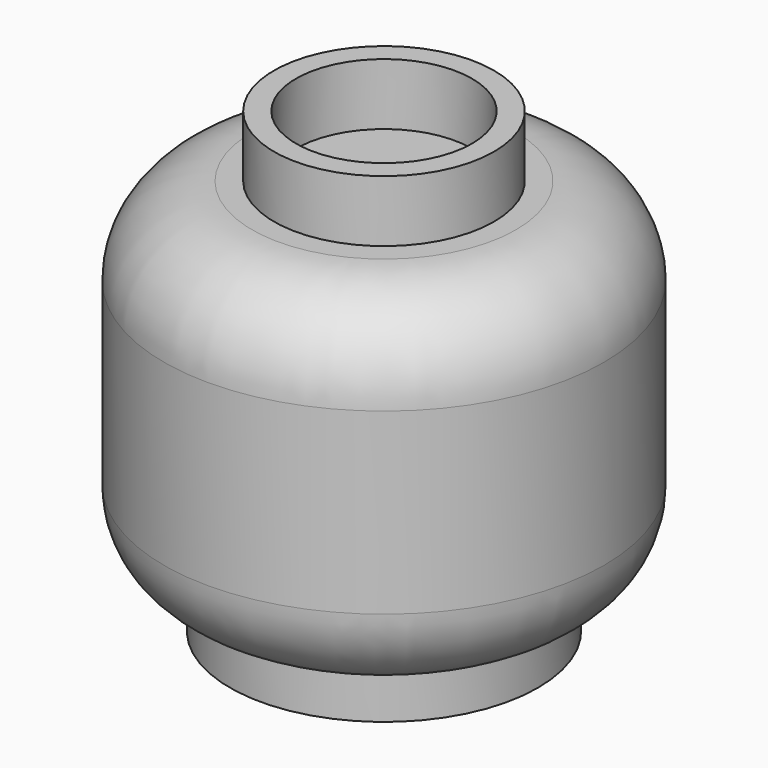
from build123d import *

# Parameters (mm, degrees)
F0_R     = 3.5
F0_R_2   = 3
F1_DEPTH = 1
F2_R     = 5
F2_R_2   = 3.5
F2_R_3   = 3
F3_DEPTH = 8
F4_R     = 2.5
F4_R_2   = 2
F5_DEPTH = 1.4
F7_DEPTH = 5


# Not quite as in the source:
# - a fillet or chamfer that OpenCascade refuses, or shapes differently, is made with other operations: its cross-section is extruded or revolved along the edge and cut away or added


with BuildPart() as f1:
    # F0 (on Top) → F1 (new body)
    with BuildSketch(Plane.XY):
        Circle(F0_R)
        Circle(F0_R_2, mode=Mode.SUBTRACT)
    extrude(amount=F1_DEPTH)

    # F2 (on face) → F3 (join)
    with BuildSketch(Plane.XY.offset(1)):
        Circle(F2_R)
        Circle(F2_R_2, mode=Mode.SUBTRACT)
        Circle(F2_R_2)
        Circle(F2_R_3, mode=Mode.SUBTRACT)
        Circle(F2_R_3)
    extrude(amount=F3_DEPTH)

    # F4 (on face) → F5 (join)
    with BuildSketch(Plane.XY.offset(9)):
        Circle(F4_R)
        Circle(F4_R_2, mode=Mode.SUBTRACT)
    extrude(amount=F5_DEPTH)

    # F6: fillet of radius 2 on 2 edges, made by hand

    # F6_s1 → F6_t2 (revolve, cut)
    with BuildSketch(Plane.XZ):
        with BuildLine():
            ThreePointArc((5, 7), (4.4142135624, 8.4142135624), (3, 9))
            Line((3, 9), (5, 9))
            Line((5, 9), (5, 7))
        make_face()
    revolve(axis=Axis((0, 0, 9), (0, 0, 1)), mode=Mode.SUBTRACT)

    # F6_s3 → F6_t4 (revolve, cut)
    with BuildSketch(Plane.XZ):
        with BuildLine():
            ThreePointArc((5, 2.9364916731), (4.5811388301, 1.7117468017), (3.5, 1))
            Line((3.5, 1), (5, 1))
            Line((5, 1), (5, 2.9364916731))
        make_face()
    revolve(axis=Axis((0, 0, 1), (0, 0, 1)), mode=Mode.SUBTRACT)

    # F7 (cut): a face of the model
    f7_faces = [f1.faces().sort_by_distance(p)[0] for p in [
        (0, 0, 1),
    ]]
    extrude(f7_faces, amount=-F7_DEPTH, mode=Mode.SUBTRACT)


solid = f1.part
